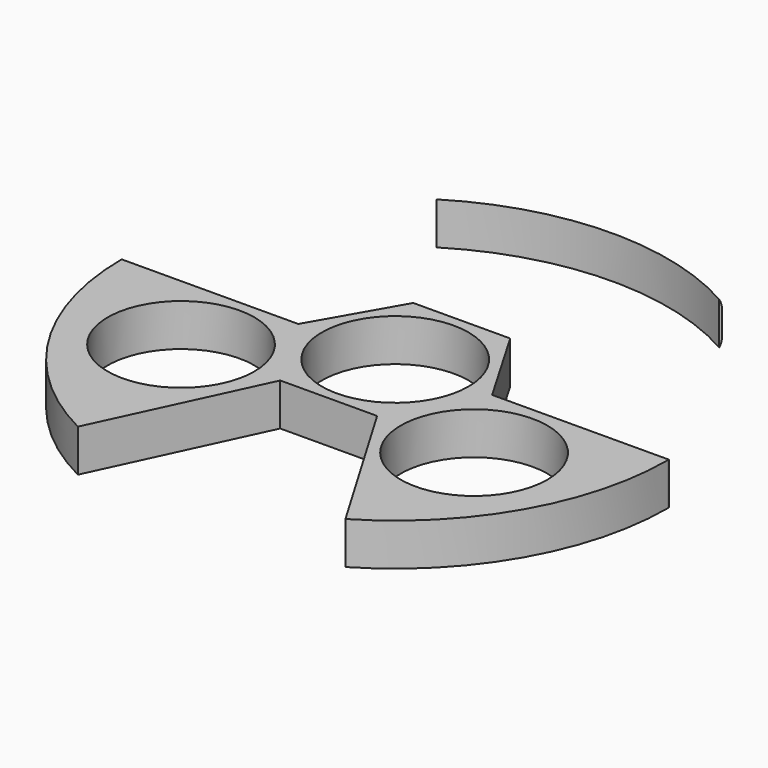
from build123d import *

# Parameters (mm, degrees)
F0_R        = 11.0109
F1_DEPTH    = 6.35
F2_T2_ANGLE = 70.1504817672
F2_T4_ANGLE = 70.1504817672


# Not quite as in the source:
# - a fillet or chamfer that OpenCascade refuses, or shapes differently, is made with other operations: its cross-section is extruded or revolved along the edge and cut away or added


with BuildPart() as f1:
    # F0 (on Top) → F1 (new body)
    with BuildSketch(Plane.XY):
        Polygon((14.4982038565, 0.0645564188), (7.1931944296, 12.5880910584), (-7.3050094269, 12.5235346396), (-14.4982038565, -0.0645564188), (-7.1931944296, -12.5880910584), (7.3050094269, -12.5235346396), align=None)
        Circle(F0_R, mode=Mode.SUBTRACT)
        with BuildLine():
            Line((-14.4982038565, -0.0645564188), (-40.9298487578, -0.1822490898))
            ThreePointArc((-40.9298487578, -0.1822490898), (-34.7949557319, -21.55450741), (-18.3913751147, -36.565599345))
            Line((-18.3913751147, -36.565599345), (-7.1931944296, -12.5880910584))
            Line((-7.1931944296, -12.5880910584), (-14.4982038565, -0.0645564188))
        make_face()
        with Locations((-21.9970452561, -12.7)):
            Circle(F0_R, mode=Mode.SUBTRACT)
        with BuildLine():
            ThreePointArc((40.9302545077, 0), (40.9301530701, 0.0911247708), (40.9298487578, 0.1822490898))
            Line((40.9298487578, 0.1822490898), (14.4982038565, 0.0645564188))
            Line((14.4982038565, 0.0645564188), (7.3050094269, -12.5235346396))
            Line((7.3050094269, -12.5235346396), (20.7483825964, -35.2815866098))
            ThreePointArc((20.7483825964, -35.2815866098), (35.5283148655, -20.3230060987), (40.9302545077, 0))
        make_face()
        with Locations((21.9970452561, -12.7)):
            Circle(F0_R, mode=Mode.SUBTRACT)
    extrude(amount=F1_DEPTH)


with BuildPart() as f1b:
    # F0 (on Top) → F1, piece 2 (new body)
    with BuildSketch(Plane.XY):
        with BuildLine():
            Line((20.1434729417, 35.6304116159), (20.3098342556, 35.9264168886))
            ThreePointArc((20.3098342556, 35.9264168886), (-0.8576214797, 41.2608929052), (-21.7851331782, 35.0514588904))
            Line((-21.7851331782, 35.0514588904), (-21.6015163476, 34.7657910244))
            ThreePointArc((-21.6015163476, 34.7657910244), (-0.8475640596, 40.921478092), (20.1434729417, 35.6304116159))
        make_face()
    extrude(amount=F1_DEPTH)

    # F2: fillet of radius 2.54 on 2 edges, made by hand

    # F2_s1 → F2_t2 (revolve, cut)
    with BuildSketch(Plane(origin=(0, 0, 0), x_dir=(0, 0, 1), z_dir=(0.8301631357, -0.5575205541, 0))):
        with BuildLine():
            ThreePointArc((1.2687086353, -41.2698049176), (0.6120283322, -41.1834493457), (0, -40.9302545077))
            Line((0, -40.9302545077), (0, -41.2698049176))
            Line((0, -41.2698049176), (1.2687086353, -41.2698049176))
        make_face()
    revolve(axis=Axis((0, 0, 0), (0, 0, 1)), revolution_arc=F2_T2_ANGLE, mode=Mode.SUBTRACT)

    # F2_s3 → F2_t4 (revolve, cut)
    with BuildSketch(Plane(origin=(0, 0, 0), x_dir=(0, 0, 1), z_dir=(0.8301631357, -0.5575205541, 0))):
        with BuildLine():
            ThreePointArc((5.0812913647, -41.2698049176), (5.7379716678, -41.1834493457), (6.35, -40.9302545077))
            Line((6.35, -40.9302545077), (6.35, -41.2698049176))
            Line((6.35, -41.2698049176), (5.0812913647, -41.2698049176))
        make_face()
    revolve(axis=Axis((0, 0, 6.35), (0, 0, 1)), revolution_arc=F2_T4_ANGLE, mode=Mode.SUBTRACT)


solid = Compound([f1.part, f1b.part])
